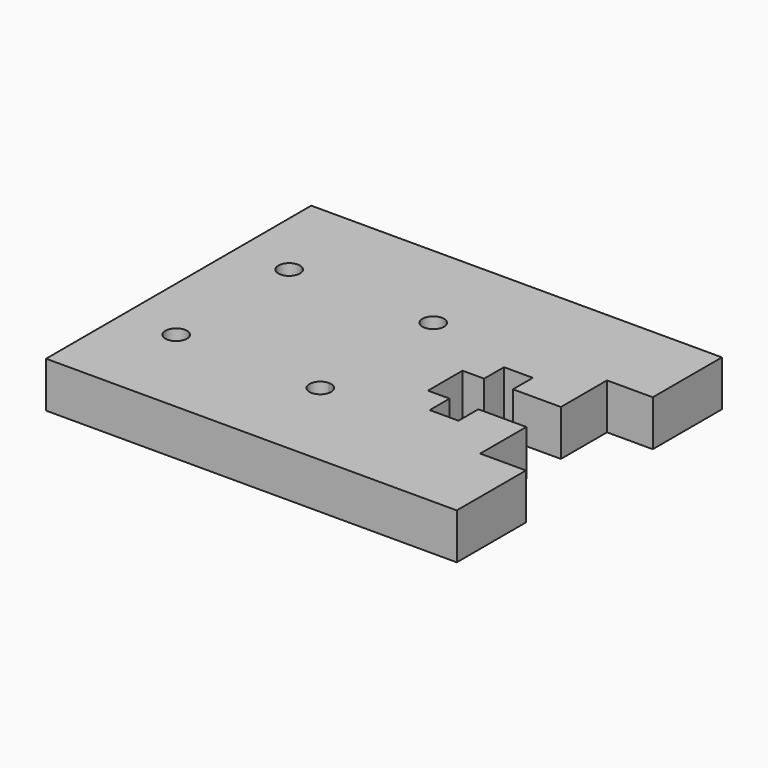
from build123d import *

# Parameters (mm, degrees)
F0_R     = 0.75
F0_W     = 3.175
F0_H     = 6
F1_DEPTH = 3.175


# Not quite as in the source:
# - a length typed as a fraction of an inch, garbled in the dataset ("3 / 203.2 mm" for 3/8 in), is restored


with BuildPart() as f1:
    # F0 (on Top) → F1 (new body)
    with BuildSketch(Plane.XY):
        Polygon((18.934352152, 7.3924250901), (18.934352152, 10.3924250901), (20.434352152, 10.3924250901), (20.434352152, 12.1162086725), (22.434352152, 12.1162086725), (22.434352152, 10.3924250901), (25.759352152, 10.3924250901), (25.759352152, 14.3924250901), (25.759352152, 20.3924250901), (0.434352152, 20.3924250901), (0.434352152, -2.6075749099), (25.759352152, -2.6075749099), (25.759352152, 3.3924250901), (25.759352152, 7.3924250901), (22.434352152, 7.3924250901), (22.434352152, 5.6686415076), (20.434352152, 5.6686415076), (20.434352152, 7.3924250901), align=None)
        with Locations((4.184352152, 3.9924250901)):
            Circle(F0_R, mode=Mode.SUBTRACT)
        with BuildLine():
            ThreePointArc((14.934352152, 3.9924250901), (13.6540220662, 3.4620950042), (14.184352152, 4.7424250901))
            ThreePointArc((14.184352152, 4.7424250901), (14.7146822379, 4.522755176), (14.934352152, 3.9924250901))
        make_face(mode=Mode.SUBTRACT)
        with Locations((4.184352152, 13.7924250901)):
            Circle(F0_R, mode=Mode.SUBTRACT)
        with BuildLine():
            ThreePointArc((14.184352152, 13.0424250901), (13.6540220662, 14.322755176), (14.934352152, 13.7924250901))
            ThreePointArc((14.934352152, 13.7924250901), (14.7146822379, 13.2620950042), (14.184352152, 13.0424250901))
        make_face(mode=Mode.SUBTRACT)
        with Locations((27.346852152, 17.3924250901)):
            Rectangle(F0_W, F0_H)
        with Locations((27.346852152, 0.3924250901)):
            Rectangle(F0_W, F0_H)
    extrude(amount=F1_DEPTH)


solid = f1.part
